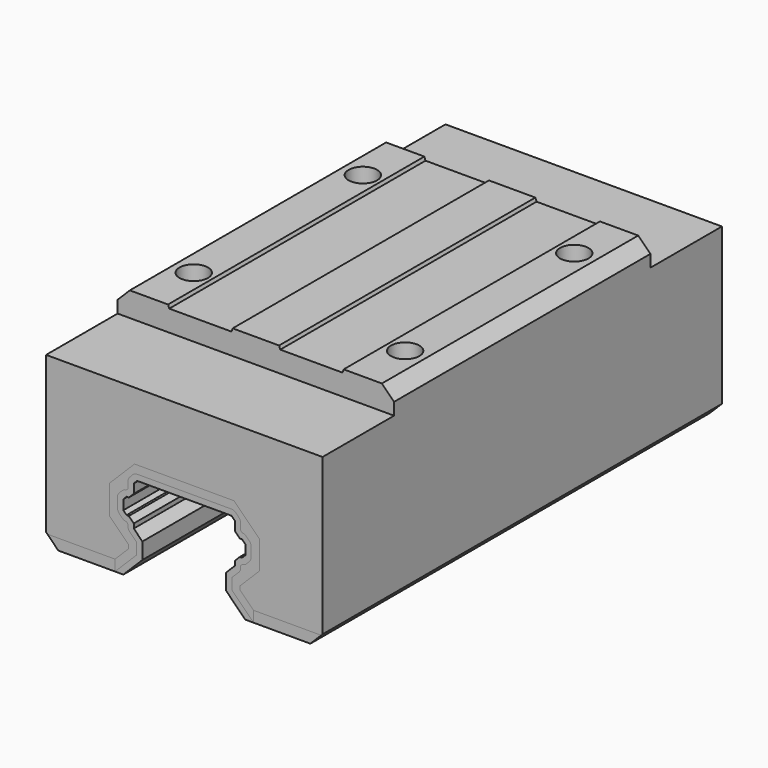
from build123d import *

# Parameters (mm, degrees)
F2_DEPTH = 30.7
F3_DEPTH = 30.7
F4_DEPTH = 30.7
F5_DEPTH = 30.7
F6_W     = 1.5
F6_H     = 11
F6_W_2   = 4.7
F6_W_3   = 27.8
F7_DEPTH = 3
F6_R     = 1.75
F8_DEPTH = 6


# Not quite as in the source:
# - ends of sketch curves that miss each other by under 0.0002 mm in the source are joined


with BuildPart() as f2:
    # F1 (on Front) → F2 (new body, symmetric)
    with BuildSketch(Plane.XZ):
        Polygon((-16.8405850499, -1.8594901503), (-8.518258067, -1.8594901503), (-6.8743992298, -0.215631313), (-6.8743992298, 0.2635278943), (-9.2200242926, 2.6091529571), (-9.2200242926, 6.1214771122), (-6.1214750979, 9.2200263069), (6.121524902, 9.2199902931), (9.2200558674, 6.1214228691), (9.2200352046, 2.6090987141), (6.8743963413, 0.2634874511), (6.8743935224, -0.2156717563), (8.5182426885, -1.8595402646), (16.8404863728, -1.8595402646), (16.9999757186, -1.7000509188), (16.9999757186, 18.9999490861), (15.4999757186, 20.4999490861), (10.7999757186, 20.4999490861), (10.6543876249, 20.0999490861), (2.9999757186, 20.0999490861), (2.8543876249, 20.4999490861), (-2.8544361877, 20.4999490861), (-3.0000242814, 20.0999490861), (-10.6544361877, 20.0999490861), (-10.8000242814, 20.4999490861), (-15.5000242814, 20.4999490861), (-17.0000242814, 18.9999490861), (-17.0000242814, -1.7000509188), align=None)
    extrude(amount=F2_DEPTH, both=True)

    # F6 (on face) → F7 (cut)
    with BuildSketch(Plane.XY.offset(20.4999490861)):
        with Locations((16.2499757186, 25.2)):
            Rectangle(F6_W, F6_H)
        with Locations((13.1499757186, 25.2)):
            Rectangle(F6_W_2, F6_H)
        with Locations((16.2499757186, -25.2)):
            Rectangle(F6_W, F6_H)
        with Locations((-3.1000242814, 25.2)):
            Rectangle(F6_W_3, F6_H)
        with Locations((13.1499757186, -25.2)):
            Rectangle(F6_W_2, F6_H)
        with Locations((-3.1000242814, -25.2)):
            Rectangle(F6_W_3, F6_H)
    extrude(amount=-F7_DEPTH, mode=Mode.SUBTRACT)

    # F6 (on face) → F8 (cut)
    with BuildSketch(Plane.XY.offset(20.4999490861)):
        with Locations((12.9999757186, 13)):
            Circle(F6_R)
        with Locations((12.9999757186, -13)):
            Circle(F6_R)
        with Locations((-13.0000242814, -13)):
            Circle(F6_R)
        with Locations((-13.0000242814, 13)):
            Circle(F6_R)
    extrude(amount=-F8_DEPTH, mode=Mode.SUBTRACT)


with BuildPart() as f3:
    # F1 (on Front) → F3 (new body, symmetric)
    with BuildSketch(Plane.XZ):
        with BuildLine():
            Line((-8.518258067, -1.8594901503), (-8.518258067, -3.2000509188))
            Line((-8.518258067, -3.2000509188), (-5.8743992298, -0.5561920816))
            Line((-5.8743992298, -0.5561920816), (-5.8743992298, 0.8473403794))
            Line((-5.8743992298, 0.8473403794), (-6.7095316198, 1.6824727694))
            ThreePointArc((-6.7095316198, 1.6824727694), (-6.8764466408, 1.9322787516), (-6.9350594016, 2.2269449988))
            Line((-6.9350594016, 2.2269449988), (-6.9350594016, 2.4600478574))
            Line((-6.9350594016, 2.4600478574), (-7.1214818731, 2.6464703778))
            ThreePointArc((-7.1214818731, 2.6464703778), (-7.3933557931, 2.7122661382), (-7.6237858327, 2.8708426413))
            Line((-7.6237858327, 2.8708426413), (-7.9944965108, 3.2415533194))
            ThreePointArc((-7.9944965108, 3.2415533194), (-8.1614115318, 3.4913593016), (-8.2200242926, 3.7860255488))
            Line((-8.2200242926, 3.7860255488), (-8.2200242926, 4.9446045204))
            ThreePointArc((-8.2200242926, 4.9446045204), (-8.1614115318, 5.2392707676), (-7.9944965108, 5.4890767499))
            Line((-7.9944965108, 5.4890767499), (-7.6237858327, 5.859787428))
            ThreePointArc((-7.6237858327, 5.859787428), (-7.3933557643, 6.0183639439), (-7.12148181, 6.0841596949))
            Line((-7.12148181, 6.0841596949), (-6.9350594016, 6.2705821033))
            Line((-6.9350594016, 6.2705821033), (-6.9350594016, 7.0585277299))
            ThreePointArc((-6.9350594016, 7.0585277299), (-6.8802359883, 7.343873925), (-6.7235725188, 7.5885872573))
            Line((-6.7235725188, 7.5885872573), (-6.3520922284, 7.9800086136))
            ThreePointArc((-6.3520922284, 7.9800086136), (-6.0975150926, 8.1574255378), (-5.7935791, 8.2199490973))
            Line((-5.7935791, 8.2199490973), (5.7935305372, 8.2199490973))
            ThreePointArc((5.7935305372, 8.2199490973), (6.0974665298, 8.1574255378), (6.3520436656, 7.9800086136))
            Line((6.3520436656, 7.9800086136), (6.723523956, 7.5885872573))
            ThreePointArc((6.723523956, 7.5885872573), (6.8801874255, 7.343873925), (6.9350108388, 7.0585277299))
            Line((6.9350108388, 7.0585277299), (6.9350108388, 6.2705821033))
            Line((6.9350108388, 6.2705821033), (7.1214332472, 6.0841596949))
            ThreePointArc((7.1214332472, 6.0841596949), (7.3933072015, 6.0183639439), (7.6237372699, 5.859787428))
            Line((7.6237372699, 5.859787428), (7.994447948, 5.4890767499))
            ThreePointArc((7.994447948, 5.4890767499), (8.161362969, 5.2392707676), (8.2199757298, 4.9446045204))
            Line((8.2199757298, 4.9446045204), (8.2199757298, 3.7860255488))
            ThreePointArc((8.2199757298, 3.7860255488), (8.161362969, 3.4913593016), (7.994447948, 3.2415533194))
            Line((7.994447948, 3.2415533194), (7.6237372699, 2.8708426413))
            ThreePointArc((7.6237372699, 2.8708426413), (7.3933072303, 2.7122661382), (7.1214333103, 2.6464703778))
            Line((7.1214333103, 2.6464703778), (6.9350108388, 2.4600478574))
            Line((6.9350108388, 2.4600478574), (6.9350108388, 2.2269449988))
            ThreePointArc((6.9350108388, 2.2269449988), (6.876398078, 1.9322787516), (6.709483057, 1.6824727694))
            Line((6.709483057, 1.6824727694), (5.874350667, 0.8473403794))
            Line((5.874350667, 0.8473403794), (5.874350667, -0.5561920816))
            Line((5.874350667, -0.5561920816), (8.5182095042, -3.2000509188))
            Line((8.5182095042, -3.2000509188), (8.5182426885, -1.8595402646))
            Line((8.5182426885, -1.8595402646), (6.8743935224, -0.2156717563))
            Line((6.8743935224, -0.2156717563), (6.8743963413, 0.2634874511))
            Line((6.8743963413, 0.2634874511), (9.2200352038, 2.6090987141))
            Line((9.2200352038, 2.6090987141), (9.2200558682, 6.1214228691))
            Line((9.2200558682, 6.1214228691), (6.121524902, 9.2199902931))
            Line((6.121524902, 9.2199902931), (-6.1214750979, 9.2200263069))
            Line((-6.1214750979, 9.2200263069), (-9.2200242926, 6.1214771122))
            Line((-9.2200242926, 6.1214771122), (-9.2200242926, 2.6091529571))
            Line((-9.2200242926, 2.6091529571), (-6.8743992298, 0.2635278943))
            Line((-6.8743992298, 0.2635278943), (-6.8743992298, -0.215631313))
            Line((-6.8743992298, -0.215631313), (-8.518258067, -1.8594901503))
        make_face()
    extrude(amount=F3_DEPTH, both=True)


with BuildPart() as f4:
    # F1 (on Front) → F4 (new body, symmetric)
    with BuildSketch(Plane.XZ):
        with BuildLine():
            Line((-8.518258067, -3.2000509188), (-7.4955332697, -3.2000509188))
            ThreePointArc((-7.4955332697, -3.2000509188), (-7.4911141393, -3.1922725839), (-7.4853796205, -3.1854062529))
            Line((-7.4853796205, -3.1854062529), (-5.1543992186, -0.8544258511))
            Line((-5.1543992186, -0.8544258511), (-5.1543992186, 1.1455741489))
            Line((-5.1543992186, 1.1455741489), (-6.2004147295, 2.1915896597))
            ThreePointArc((-6.2004147295, 2.1915896597), (-6.211253367, 2.2078108272), (-6.2150593904, 2.2269449988))
            Line((-6.2150593904, 2.2269449988), (-6.2150593904, 2.7582815716))
            Line((-6.2150593904, 2.7582815716), (-6.8220925303, 3.3653148707))
            Line((-6.8220925303, 3.3653148707), (-7.0793136033, 3.3653148707))
            ThreePointArc((-7.0793136033, 3.3653148707), (-7.0984477749, 3.3691208941), (-7.1146689424, 3.3799595317))
            Line((-7.1146689424, 3.3799595317), (-7.4853796205, 3.7506702098))
            ThreePointArc((-7.4853796205, 3.7506702098), (-7.496218258, 3.7668913772), (-7.5000242814, 3.7860255488))
            Line((-7.5000242814, 3.7860255488), (-7.5000242814, 4.9446045204))
            ThreePointArc((-7.5000242814, 4.9446045204), (-7.496218258, 4.9637386921), (-7.4853796205, 4.9799598595))
            Line((-7.4853796205, 4.9799598595), (-7.1146689424, 5.3506705376))
            ThreePointArc((-7.1146689424, 5.3506705376), (-7.0984477749, 5.3615091752), (-7.0793136033, 5.3653151986))
            Line((-7.0793136033, 5.3653151986), (-6.8220925256, 5.3653151986))
            Line((-6.8220925256, 5.3653151986), (-6.2150593904, 5.9723483338))
            Line((-6.2150593904, 5.9723483338), (-6.2150593904, 7.0585277299))
            ThreePointArc((-6.2150593904, 7.0585277299), (-6.2114994286, 7.0770567033), (-6.2013264761, 7.0929471792))
            Line((-6.2013264761, 7.0929471792), (-5.8298461857, 7.4843685354))
            ThreePointArc((-5.8298461857, 7.4843685354), (-5.8133152031, 7.4958891148), (-5.7935791, 7.4999490861))
            Line((-5.7935791, 7.4999490861), (5.7935305372, 7.4999490861))
            ThreePointArc((5.7935305372, 7.4999490861), (5.8132666403, 7.4958891148), (5.8297976229, 7.4843685354))
            Line((5.8297976229, 7.4843685354), (6.2012779133, 7.0929471792))
            ThreePointArc((6.2012779133, 7.0929471792), (6.2114508657, 7.0770567033), (6.2150108276, 7.0585277299))
            Line((6.2150108276, 7.0585277299), (6.2150108276, 5.9723483338))
            Line((6.2150108276, 5.9723483338), (6.8220439628, 5.3653151986))
            Line((6.8220439628, 5.3653151986), (7.0792650405, 5.3653151986))
            ThreePointArc((7.0792650405, 5.3653151986), (7.0983992121, 5.3615091752), (7.1146203795, 5.3506705376))
            Line((7.1146203795, 5.3506705376), (7.4853310576, 4.9799598595))
            ThreePointArc((7.4853310576, 4.9799598595), (7.4961696952, 4.9637386921), (7.4999757186, 4.9446045204))
            Line((7.4999757186, 4.9446045204), (7.4999757186, 3.7860255488))
            ThreePointArc((7.4999757186, 3.7860255488), (7.4961696952, 3.7668913772), (7.4853310576, 3.7506702098))
            Line((7.4853310576, 3.7506702098), (7.1146203795, 3.3799595317))
            ThreePointArc((7.1146203795, 3.3799595317), (7.0983992121, 3.3691208941), (7.0792650405, 3.3653148707))
            Line((7.0792650405, 3.3653148707), (6.8220439674, 3.3653148707))
            Line((6.8220439674, 3.3653148707), (6.2150108276, 2.7582815716))
            Line((6.2150108276, 2.7582815716), (6.2150108276, 2.2269449988))
            ThreePointArc((6.2150108276, 2.2269449988), (6.2112048042, 2.2078108272), (6.2003661666, 2.1915896597))
            Line((6.2003661666, 2.1915896597), (5.1543506558, 1.1455741489))
            Line((5.1543506558, 1.1455741489), (5.1543506558, -0.8544258511))
            Line((5.1543506558, -0.8544258511), (7.4853310576, -3.1854062529))
            ThreePointArc((7.4853310576, -3.1854062529), (7.4910835469, -3.1922985202), (7.4955108104, -3.2001083741))
            Line((7.4955108104, -3.2001083741), (8.5182221531, -3.2001010332))
            Line((8.5182221531, -3.2001010332), (5.874350667, -0.5561920816))
            Line((5.874350667, -0.5561920816), (5.874350667, 0.8473403794))
            Line((5.874350667, 0.8473403794), (6.709483057, 1.6824727694))
            ThreePointArc((6.709483057, 1.6824727694), (6.876398078, 1.9322787516), (6.9350108388, 2.2269449988))
            Line((6.9350108388, 2.2269449988), (6.9350108388, 2.4600478574))
            Line((6.9350108388, 2.4600478574), (7.1214333103, 2.6464703778))
            ThreePointArc((7.1214333103, 2.6464703778), (7.3933072303, 2.7122661382), (7.6237372699, 2.8708426413))
            Line((7.6237372699, 2.8708426413), (7.994447948, 3.2415533194))
            ThreePointArc((7.994447948, 3.2415533194), (8.161362969, 3.4913593016), (8.2199757298, 3.7860255488))
            Line((8.2199757298, 3.7860255488), (8.2199757298, 4.9446045204))
            ThreePointArc((8.2199757298, 4.9446045204), (8.161362969, 5.2392707676), (7.994447948, 5.4890767499))
            Line((7.994447948, 5.4890767499), (7.6237372699, 5.859787428))
            ThreePointArc((7.6237372699, 5.859787428), (7.3933072015, 6.0183639439), (7.1214332472, 6.0841596949))
            Line((7.1214332472, 6.0841596949), (6.9350108388, 6.2705821033))
            Line((6.9350108388, 6.2705821033), (6.9350108388, 7.0585277299))
            ThreePointArc((6.9350108388, 7.0585277299), (6.8801874255, 7.343873925), (6.723523956, 7.5885872573))
            Line((6.723523956, 7.5885872573), (6.3520436656, 7.9800086136))
            ThreePointArc((6.3520436656, 7.9800086136), (6.0974665298, 8.1574255378), (5.7935305372, 8.2199490973))
            Line((5.7935305372, 8.2199490973), (-5.7935791, 8.2199490973))
            ThreePointArc((-5.7935791, 8.2199490973), (-6.0975150926, 8.1574255378), (-6.3520922284, 7.9800086136))
            Line((-6.3520922284, 7.9800086136), (-6.7235725188, 7.5885872573))
            ThreePointArc((-6.7235725188, 7.5885872573), (-6.8802359883, 7.343873925), (-6.9350594016, 7.0585277299))
            Line((-6.9350594016, 7.0585277299), (-6.9350594016, 6.2705821033))
            Line((-6.9350594016, 6.2705821033), (-7.12148181, 6.0841596949))
            ThreePointArc((-7.12148181, 6.0841596949), (-7.3933557643, 6.0183639439), (-7.6237858327, 5.859787428))
            Line((-7.6237858327, 5.859787428), (-7.9944965108, 5.4890767499))
            ThreePointArc((-7.9944965108, 5.4890767499), (-8.1614115318, 5.2392707676), (-8.2200242926, 4.9446045204))
            Line((-8.2200242926, 4.9446045204), (-8.2200242926, 3.7860255488))
            ThreePointArc((-8.2200242926, 3.7860255488), (-8.1614115318, 3.4913593016), (-7.9944965108, 3.2415533194))
            Line((-7.9944965108, 3.2415533194), (-7.6237858327, 2.8708426413))
            ThreePointArc((-7.6237858327, 2.8708426413), (-7.3933557931, 2.7122661382), (-7.1214818731, 2.6464703778))
            Line((-7.1214818731, 2.6464703778), (-6.9350594016, 2.4600478574))
            Line((-6.9350594016, 2.4600478574), (-6.9350594016, 2.2269449988))
            ThreePointArc((-6.9350594016, 2.2269449988), (-6.8764466408, 1.9322787516), (-6.7095316198, 1.6824727694))
            Line((-6.7095316198, 1.6824727694), (-5.8743992298, 0.8473403794))
            Line((-5.8743992298, 0.8473403794), (-5.8743992298, -0.5561920816))
            Line((-5.8743992298, -0.5561920816), (-8.518258067, -3.2000509188))
        make_face()
    extrude(amount=F4_DEPTH, both=True)


with BuildPart() as f5:
    # F1 (on Front) → F5 (new body, symmetric)
    with BuildSketch(Plane.XZ):
        Polygon((-15.5000242814, -3.2000509188), (-8.518258067, -3.2000509188), (-8.518258067, -1.8594901503), (-16.8405850499, -1.8594901503), align=None)
    extrude(amount=F5_DEPTH, both=True)


with BuildPart() as f5b:
    # F1 (on Front) → F5, piece 2 (new body, symmetric)
    with BuildSketch(Plane.XZ):
        Polygon((8.5182426885, -1.8595402646), (8.5182348017, -3.2001010331), (15.4999757186, -3.2000509188), (16.8404863728, -1.8595402646), align=None)
    extrude(amount=F5_DEPTH, both=True)


solid = Compound([f2.part, f3.part, f4.part, f5.part, f5b.part])
